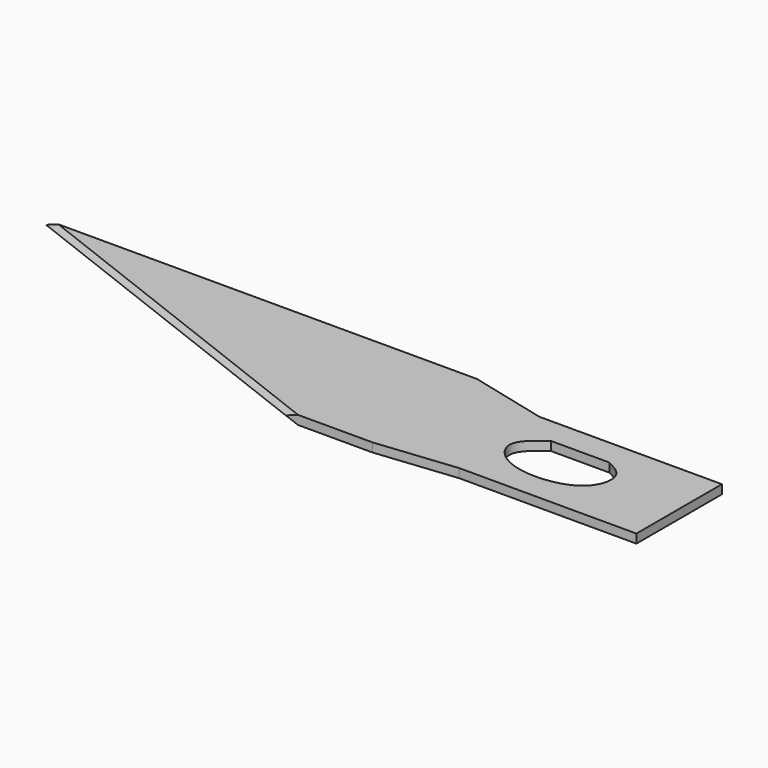
from build123d import *

# Parameters (mm, degrees)
F1_DEPTH    = 0.5
F2_T1_DEPTH = 24.3877615645


# Not quite as in the source:
# - a fillet or chamfer that OpenCascade refuses, or shapes differently, is made with other operations: its cross-section is extruded or revolved along the edge and cut away or added


with BuildPart() as f1:
    # F0 (on Top) → F1 (new body)
    with BuildSketch(Plane.XY):
        Polygon((12.5838547959, -11.2850121383), (-12.2901993096, -11.2850121383), (7.2110601937, -18.846724632), (12.7828468132, -18.846724632), (17.260177021, -18.3794706089), (27.2098006904, -18.3794706089), (27.2098006904, -12.3794706089), (16.9616886783, -12.3794706089), align=None)
        with BuildLine():
            add(Edge.make_bspline(
                [(22.0857446844, -13.8540112255), (22.5057904818, -14.0714719098), (23.4075383771, -14.5383131818), (22.856226593, -16.8955850574), (18.716199205, -17.1776625989), (17.0863515211, -15.1231779615), (18.2240211185, -14.2724034673), (18.7835020814, -13.8540112255)],
                knots=[0, 0, 0, 0, 0.1610304719, 0.3456977548, 0.6171279231, 0.8117119076, 1, 1, 1, 1], degree=3))
            Line((18.7835020814, -13.8540112255), (22.0857446844, -13.8540112255))
        make_face(mode=Mode.SUBTRACT)
    extrude(amount=F1_DEPTH)

    # F2: chamfer of 0.5 on 2 edges, made by hand

    # F2_s2 → F2_t1 (cut)
    with BuildSketch(Plane(origin=(-8.0788192676, 3.1326032342, 0), x_dir=(0, 0, 1), z_dir=(0.932361315, -0.3615278389, 0))):
        Polygon((0, 14.9649579531), (0.5, 14.4649579531), (0.5, 14.9649579531), align=None)
        Polygon((0.5, 14.9649579531), (0, 14.4649579531), (0, 14.9649579531), align=None)
    extrude(amount=F2_T1_DEPTH, mode=Mode.SUBTRACT)


solid = f1.part
